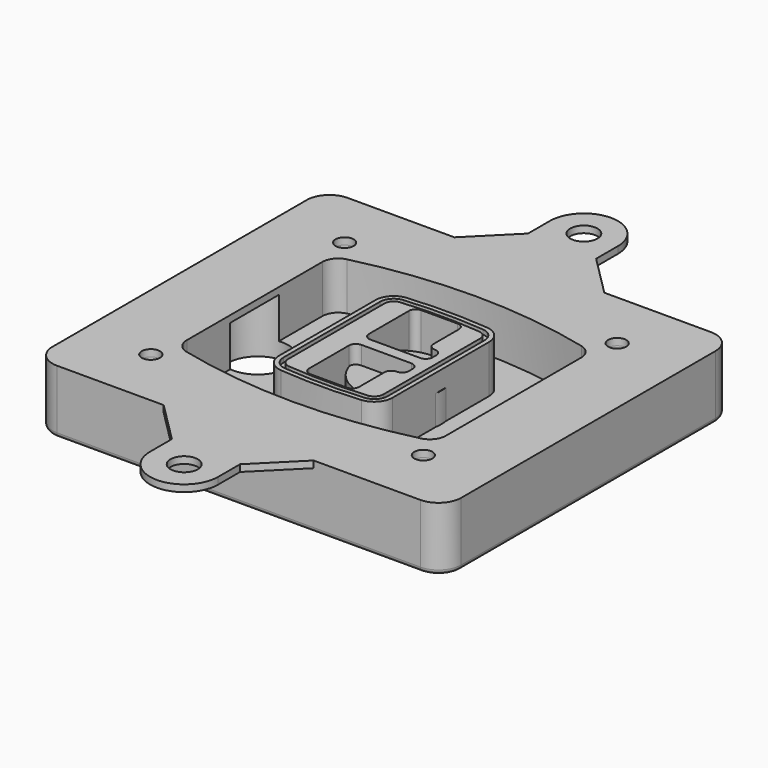
from build123d import *

# Parameters (mm, degrees)
F0_R      = 4
F1_DEPTH  = 25
F2_DEPTH  = 3
F3_DEPTH  = 18
F5_DEPTH  = 21
F6_DEPTH  = 2
F8_DEPTH  = 20
F9_DEPTH  = 16
F10_DEPTH = 25
F7_R      = 6
F7_R_2    = 4
F11_DEPTH = 6
F13_DEPTH = 9
F15_R     = 2
F16_R     = 4
F16_R_2   = 6
F17_DEPTH = 3


# Not quite as in the source:
# - a feature of the source that left no trace in its solid (it failed there, or was rolled back) is left out
# - a feature names something its author has since deleted; it is built from what else it names


with BuildPart() as f1:
    # F0 (on Top) → F1 (new body)
    with BuildSketch(Plane.XY):
        with BuildLine():
            ThreePointArc((-90, -70), (-87.0710678119, -77.0710678119), (-80, -80))
            Line((-80, -80), (80, -80))
            ThreePointArc((80, -80), (87.0710678119, -77.0710678119), (90, -70))
            Line((90, -70), (90, 70))
            ThreePointArc((90, 70), (87.0710678119, 77.0710678119), (80, 80))
            Line((80, 80), (-80, 80))
            ThreePointArc((-80, 80), (-87.0710678119, 77.0710678119), (-90, 70))
            Line((-90, 70), (-90, -70))
        make_face()
        with Locations((-60, -53.3333333333)):
            Circle(F0_R, mode=Mode.SUBTRACT)
        with Locations((60, -53.3333333333)):
            Circle(F0_R, mode=Mode.SUBTRACT)
        with Locations((-60, 53.3333333333)):
            Circle(F0_R, mode=Mode.SUBTRACT)
        with BuildLine():
            ThreePointArc((-64, 37.2990447398), (-61.0143011354, 45.9411029726), (-53.3306899286, 50.8970778549))
            ThreePointArc((-53.3306899286, 50.8970778549), (0, 57.3333333333), (53.3306899286, 50.8970778549))
            ThreePointArc((53.3306899286, 50.8970778549), (61.0143011354, 45.9411029726), (64, 37.2990447398))
            Line((64, 37.2990447398), (64, -37.2990447398))
            ThreePointArc((64, -37.2990447398), (61.0143011354, -45.9411029726), (53.3306899286, -50.8970778549))
            ThreePointArc((53.3306899286, -50.8970778549), (0, -57.3333333333), (-53.3306899286, -50.8970778549))
            ThreePointArc((-53.3306899286, -50.8970778549), (-61.0143011354, -45.9411029726), (-64, -37.2990447398))
            Line((-64, -37.2990447398), (-64, 37.2990447398))
        make_face(mode=Mode.SUBTRACT)
        with Locations((60, 53.3333333333)):
            Circle(F0_R, mode=Mode.SUBTRACT)
        with BuildLine():
            ThreePointArc((53.3306899286, 50.8970778549), (0, 57.3333333333), (-53.3306899286, 50.8970778549))
            ThreePointArc((-53.3306899286, 50.8970778549), (-61.0143011354, 45.9411029726), (-64, 37.2990447398))
            Line((-64, 37.2990447398), (-64, -37.2990447398))
            ThreePointArc((-64, -37.2990447398), (-61.0143011354, -45.9411029726), (-53.3306899286, -50.8970778549))
            ThreePointArc((-53.3306899286, -50.8970778549), (0, -57.3333333333), (53.3306899286, -50.8970778549))
            ThreePointArc((53.3306899286, -50.8970778549), (61.0143011354, -45.9411029726), (64, -37.2990447398))
            Line((64, -37.2990447398), (64, 37.2990447398))
            ThreePointArc((64, 37.2990447398), (61.0143011354, 45.9411029726), (53.3306899286, 50.8970778549))
        make_face()
        with BuildLine():
            Line((-60, -37.2990447398), (-60, 37.2990447398))
            ThreePointArc((-60, 37.2990447398), (-57.8673579538, 43.4719434775), (-52.3790642347, 47.0119255363))
            ThreePointArc((-52.3790642347, 47.0119255363), (0, 53.3333333333), (52.3790642347, 47.0119255363))
            ThreePointArc((52.3790642347, 47.0119255363), (57.8673579538, 43.4719434775), (60, 37.2990447398))
            Line((60, 37.2990447398), (60, -37.2990447398))
            ThreePointArc((60, -37.2990447398), (57.8673579538, -43.4719434775), (52.3790642347, -47.0119255363))
            ThreePointArc((52.3790642347, -47.0119255363), (0, -53.3333333333), (-52.3790642347, -47.0119255363))
            ThreePointArc((-52.3790642347, -47.0119255363), (-57.8673579538, -43.4719434775), (-60, -37.2990447398))
        make_face(mode=Mode.SUBTRACT)
        with BuildLine():
            ThreePointArc((-52.3790642347, 47.0119255363), (-57.8673579538, 43.4719434775), (-60, 37.2990447398))
            Line((-60, 37.2990447398), (-60, -37.2990447398))
            ThreePointArc((-60, -37.2990447398), (-57.8673579538, -43.4719434775), (-52.3790642347, -47.0119255363))
            ThreePointArc((-52.3790642347, -47.0119255363), (0, -53.3333333333), (52.3790642347, -47.0119255363))
            ThreePointArc((52.3790642347, -47.0119255363), (57.8673579538, -43.4719434775), (60, -37.2990447398))
            Line((60, -37.2990447398), (60, 37.2990447398))
            ThreePointArc((60, 37.2990447398), (57.8673579538, 43.4719434775), (52.3790642347, 47.0119255363))
            ThreePointArc((52.3790642347, 47.0119255363), (0, 53.3333333333), (-52.3790642347, 47.0119255363))
        make_face()
        with BuildLine():
            ThreePointArc((51.6653449643, 44.0980612973), (55.5071505677, 41.6200738562), (57, 37.2990447398))
            Line((57, 37.2990447398), (57, -37.2990447398))
            ThreePointArc((57, -37.2990447398), (55.5071505677, -41.6200738562), (51.6653449643, -44.0980612973))
            ThreePointArc((51.6653449643, -44.0980612973), (0, -50.3333333333), (-51.6653449643, -44.0980612973))
            ThreePointArc((-51.6653449643, -44.0980612973), (-55.5071505677, -41.6200738562), (-57, -37.2990447398))
            Line((-57, -37.2990447398), (-57, 37.2990447398))
            ThreePointArc((-57, 37.2990447398), (-55.5071505677, 41.6200738562), (-51.6653449643, 44.0980612973))
            ThreePointArc((-51.6653449643, 44.0980612973), (0, 50.3333333333), (51.6653449643, 44.0980612973))
        make_face(mode=Mode.SUBTRACT)
        with BuildLine():
            Line((57, -37.2990447398), (57, 37.2990447398))
            ThreePointArc((57, 37.2990447398), (55.5071505677, 41.6200738562), (51.6653449643, 44.0980612973))
            ThreePointArc((51.6653449643, 44.0980612973), (0, 50.3333333333), (-51.6653449643, 44.0980612973))
            ThreePointArc((-51.6653449643, 44.0980612973), (-55.5071505677, 41.6200738562), (-57, 37.2990447398))
            Line((-57, 37.2990447398), (-57, -37.2990447398))
            ThreePointArc((-57, -37.2990447398), (-55.5071505677, -41.6200738562), (-51.6653449643, -44.0980612973))
            ThreePointArc((-51.6653449643, -44.0980612973), (0, -50.3333333333), (51.6653449643, -44.0980612973))
            ThreePointArc((51.6653449643, -44.0980612973), (55.5071505677, -41.6200738562), (57, -37.2990447398))
        make_face()
    extrude(amount=-F1_DEPTH)

    # F0 (on Top) → F2 (join)
    with BuildSketch(Plane.XY):
        with BuildLine():
            ThreePointArc((-52.3790642347, 47.0119255363), (-57.8673579538, 43.4719434775), (-60, 37.2990447398))
            Line((-60, 37.2990447398), (-60, -37.2990447398))
            ThreePointArc((-60, -37.2990447398), (-57.8673579538, -43.4719434775), (-52.3790642347, -47.0119255363))
            ThreePointArc((-52.3790642347, -47.0119255363), (0, -53.3333333333), (52.3790642347, -47.0119255363))
            ThreePointArc((52.3790642347, -47.0119255363), (57.8673579538, -43.4719434775), (60, -37.2990447398))
            Line((60, -37.2990447398), (60, 37.2990447398))
            ThreePointArc((60, 37.2990447398), (57.8673579538, 43.4719434775), (52.3790642347, 47.0119255363))
            ThreePointArc((52.3790642347, 47.0119255363), (0, 53.3333333333), (-52.3790642347, 47.0119255363))
        make_face()
        with BuildLine():
            ThreePointArc((51.6653449643, 44.0980612973), (55.5071505677, 41.6200738562), (57, 37.2990447398))
            Line((57, 37.2990447398), (57, -37.2990447398))
            ThreePointArc((57, -37.2990447398), (55.5071505677, -41.6200738562), (51.6653449643, -44.0980612973))
            ThreePointArc((51.6653449643, -44.0980612973), (0, -50.3333333333), (-51.6653449643, -44.0980612973))
            ThreePointArc((-51.6653449643, -44.0980612973), (-55.5071505677, -41.6200738562), (-57, -37.2990447398))
            Line((-57, -37.2990447398), (-57, 37.2990447398))
            ThreePointArc((-57, 37.2990447398), (-55.5071505677, 41.6200738562), (-51.6653449643, 44.0980612973))
            ThreePointArc((-51.6653449643, 44.0980612973), (0, 50.3333333333), (51.6653449643, 44.0980612973))
        make_face(mode=Mode.SUBTRACT)
    extrude(amount=F2_DEPTH)

    # F0 (on Top) → F3 (cut)
    with BuildSketch(Plane.XY):
        with BuildLine():
            Line((57, -37.2990447398), (57, 37.2990447398))
            ThreePointArc((57, 37.2990447398), (55.5071505677, 41.6200738562), (51.6653449643, 44.0980612973))
            ThreePointArc((51.6653449643, 44.0980612973), (0, 50.3333333333), (-51.6653449643, 44.0980612973))
            ThreePointArc((-51.6653449643, 44.0980612973), (-55.5071505677, 41.6200738562), (-57, 37.2990447398))
            Line((-57, 37.2990447398), (-57, -37.2990447398))
            ThreePointArc((-57, -37.2990447398), (-55.5071505677, -41.6200738562), (-51.6653449643, -44.0980612973))
            ThreePointArc((-51.6653449643, -44.0980612973), (0, -50.3333333333), (51.6653449643, -44.0980612973))
            ThreePointArc((51.6653449643, -44.0980612973), (55.5071505677, -41.6200738562), (57, -37.2990447398))
        make_face()
    extrude(amount=-F3_DEPTH, mode=Mode.SUBTRACT)

    # F4 (on face) → F5 (join, through all)
    with BuildSketch(Plane.XY.offset(3)):
        with BuildLine():
            ThreePointArc((-25, -26.587695628), (-22.8992979869, -31.9912392117), (-17.7004291845, -34.5569740744))
            ThreePointArc((-17.7004291845, -34.5569740744), (0, -35.3333333333), (17.7004291845, -34.5569740744))
            ThreePointArc((17.7004291845, -34.5569740744), (22.8992979869, -31.9912392117), (25, -26.587695628))
            Line((25, -26.587695628), (25, 26.587695628))
            ThreePointArc((25, 26.587695628), (22.8992979869, 31.9912392117), (17.7004291845, 34.5569740744))
            ThreePointArc((17.7004291845, 34.5569740744), (0, 35.3333333333), (-17.7004291845, 34.5569740744))
            ThreePointArc((-17.7004291845, 34.5569740744), (-22.8992979869, 31.9912392117), (-25, 26.587695628))
            Line((-25, 26.587695628), (-25, -26.587695628))
        make_face()
        with BuildLine():
            ThreePointArc((17.5253218884, 32.5646544628), (21.4244734902, 30.6403533158), (23, 26.587695628))
            Line((23, 26.587695628), (23, -26.587695628))
            ThreePointArc((23, -26.587695628), (21.4244734902, -30.6403533158), (17.5253218884, -32.5646544628))
            ThreePointArc((17.5253218884, -32.5646544628), (0, -33.3333333333), (-17.5253218884, -32.5646544628))
            ThreePointArc((-17.5253218884, -32.5646544628), (-21.4244734902, -30.6403533158), (-23, -26.587695628))
            Line((-23, -26.587695628), (-23, 26.587695628))
            ThreePointArc((-23, 26.587695628), (-21.4244734902, 30.6403533158), (-17.5253218884, 32.5646544628))
            ThreePointArc((-17.5253218884, 32.5646544628), (0, 33.3333333333), (17.5253218884, 32.5646544628))
        make_face(mode=Mode.SUBTRACT)
        with BuildLine():
            Line((23, -26.587695628), (23, 26.587695628))
            ThreePointArc((23, 26.587695628), (21.4244734902, 30.6403533158), (17.5253218884, 32.5646544628))
            ThreePointArc((17.5253218884, 32.5646544628), (0, 33.3333333333), (-17.5253218884, 32.5646544628))
            ThreePointArc((-17.5253218884, 32.5646544628), (-21.4244734902, 30.6403533158), (-23, 26.587695628))
            Line((-23, 26.587695628), (-23, -26.587695628))
            ThreePointArc((-23, -26.587695628), (-21.4244734902, -30.6403533158), (-17.5253218884, -32.5646544628))
            ThreePointArc((-17.5253218884, -32.5646544628), (0, -33.3333333333), (17.5253218884, -32.5646544628))
            ThreePointArc((17.5253218884, -32.5646544628), (21.4244734902, -30.6403533158), (23, -26.587695628))
        make_face()
        with BuildLine():
            ThreePointArc((17.3502145923, 30.5723348512), (19.9496489934, 29.2894674198), (21, 26.587695628))
            Line((21, 26.587695628), (21, -26.587695628))
            ThreePointArc((21, -26.587695628), (19.9496489934, -29.2894674198), (17.3502145923, -30.5723348512))
            ThreePointArc((17.3502145923, -30.5723348512), (0, -31.3333333333), (-17.3502145923, -30.5723348512))
            ThreePointArc((-17.3502145923, -30.5723348512), (-19.9496489934, -29.2894674198), (-21, -26.587695628))
            Line((-21, -26.587695628), (-21, 26.587695628))
            ThreePointArc((-21, 26.587695628), (-19.9496489934, 29.2894674198), (-17.3502145923, 30.5723348512))
            ThreePointArc((-17.3502145923, 30.5723348512), (0, 31.3333333333), (17.3502145923, 30.5723348512))
        make_face(mode=Mode.SUBTRACT)
        with BuildLine():
            Line((21, -26.587695628), (21, 26.587695628))
            ThreePointArc((21, 26.587695628), (19.9496489934, 29.2894674198), (17.3502145923, 30.5723348512))
            ThreePointArc((17.3502145923, 30.5723348512), (0, 31.3333333333), (-17.3502145923, 30.5723348512))
            ThreePointArc((-17.3502145923, 30.5723348512), (-19.9496489934, 29.2894674198), (-21, 26.587695628))
            Line((-21, 26.587695628), (-21, -26.587695628))
            ThreePointArc((-21, -26.587695628), (-19.9496489934, -29.2894674198), (-17.3502145923, -30.5723348512))
            ThreePointArc((-17.3502145923, -30.5723348512), (0, -31.3333333333), (17.3502145923, -30.5723348512))
            ThreePointArc((17.3502145923, -30.5723348512), (19.9496489934, -29.2894674198), (21, -26.587695628))
        make_face()
        with BuildLine():
            Line((-8, -2.5), (14, -2.5))
            ThreePointArc((14, -2.5), (16.1213203436, -3.3786796564), (17, -5.5))
            Line((17, -5.5), (17, -7.5))
            ThreePointArc((17, -7.5), (16.1213203436, -9.6213203436), (14, -10.5))
            ThreePointArc((14, -10.5), (11.8786796564, -11.3786796564), (11, -13.5))
            Line((11, -13.5), (11, -27.5))
            ThreePointArc((11, -27.5), (10.1213203436, -29.6213203436), (8, -30.5))
            Line((8, -30.5), (-8, -30.5))
            ThreePointArc((-8, -30.5), (-10.1213203436, -29.6213203436), (-11, -27.5))
            Line((-11, -27.5), (-11, -5.5))
            ThreePointArc((-11, -5.5), (-10.1213203436, -3.3786796564), (-8, -2.5))
        make_face(mode=Mode.SUBTRACT)
        with BuildLine():
            ThreePointArc((-8, 2.5), (-10.1213203436, 3.3786796564), (-11, 5.5))
            Line((-11, 5.5), (-11, 27.5))
            ThreePointArc((-11, 27.5), (-10.1213203436, 29.6213203436), (-8, 30.5))
            Line((-8, 30.5), (8, 30.5))
            ThreePointArc((8, 30.5), (10.1213203436, 29.6213203436), (11, 27.5))
            Line((11, 27.5), (11, 13.5))
            ThreePointArc((11, 13.5), (11.8786796564, 11.3786796564), (14, 10.5))
            ThreePointArc((14, 10.5), (16.1213203436, 9.6213203436), (17, 7.5))
            Line((17, 7.5), (17, 5.5))
            ThreePointArc((17, 5.5), (16.1213203436, 3.3786796564), (14, 2.5))
            Line((14, 2.5), (-8, 2.5))
        make_face(mode=Mode.SUBTRACT)
    extrude(amount=-F5_DEPTH)

    # F4 (on face) → F6 (cut)
    with BuildSketch(Plane.XY.offset(3)):
        with BuildLine():
            Line((23, -26.587695628), (23, 26.587695628))
            ThreePointArc((23, 26.587695628), (21.4244734902, 30.6403533158), (17.5253218884, 32.5646544628))
            ThreePointArc((17.5253218884, 32.5646544628), (0, 33.3333333333), (-17.5253218884, 32.5646544628))
            ThreePointArc((-17.5253218884, 32.5646544628), (-21.4244734902, 30.6403533158), (-23, 26.587695628))
            Line((-23, 26.587695628), (-23, -26.587695628))
            ThreePointArc((-23, -26.587695628), (-21.4244734902, -30.6403533158), (-17.5253218884, -32.5646544628))
            ThreePointArc((-17.5253218884, -32.5646544628), (0, -33.3333333333), (17.5253218884, -32.5646544628))
            ThreePointArc((17.5253218884, -32.5646544628), (21.4244734902, -30.6403533158), (23, -26.587695628))
        make_face()
        with BuildLine():
            ThreePointArc((17.3502145923, 30.5723348512), (19.9496489934, 29.2894674198), (21, 26.587695628))
            Line((21, 26.587695628), (21, -26.587695628))
            ThreePointArc((21, -26.587695628), (19.9496489934, -29.2894674198), (17.3502145923, -30.5723348512))
            ThreePointArc((17.3502145923, -30.5723348512), (0, -31.3333333333), (-17.3502145923, -30.5723348512))
            ThreePointArc((-17.3502145923, -30.5723348512), (-19.9496489934, -29.2894674198), (-21, -26.587695628))
            Line((-21, -26.587695628), (-21, 26.587695628))
            ThreePointArc((-21, 26.587695628), (-19.9496489934, 29.2894674198), (-17.3502145923, 30.5723348512))
            ThreePointArc((-17.3502145923, 30.5723348512), (0, 31.3333333333), (17.3502145923, 30.5723348512))
        make_face(mode=Mode.SUBTRACT)
    extrude(amount=-F6_DEPTH, mode=Mode.SUBTRACT)

    # F7 (on face) → F8 (join)
    with BuildSketch(Plane(origin=(0, 0, -25), x_dir=(1, 0, 0), z_dir=(0, 0, -1))):
        with BuildLine():
            ThreePointArc((-6.71157564, 0), (6.7567035675, 13.4682792075), (20.224982775, 0))
            Line((20.224982775, 0), (25.224982775, 0))
            ThreePointArc((25.224982775, 0), (6.7567035675, 18.4682792075), (-11.71157564, 0))
            Line((-11.71157564, 0), (-6.71157564, 0))
        make_face()
        with BuildLine():
            Line((-6.71157564, 0), (20.224982775, 0))
            ThreePointArc((20.224982775, 0), (6.7567035675, 13.4682792075), (-6.71157564, 0))
        make_face()
        with BuildLine():
            ThreePointArc((-6.71157564, 0), (6.7567035675, -13.4682792075), (20.224982775, 0))
            Line((20.224982775, 0), (-6.71157564, 0))
        make_face()
        with BuildLine():
            Line((25.224982775, 0), (20.224982775, 0))
            ThreePointArc((20.224982775, 0), (6.7567035675, -13.4682792075), (-6.71157564, 0))
            Line((-6.71157564, 0), (-11.71157564, 0))
            ThreePointArc((-11.71157564, 0), (6.7567035675, -18.4682792075), (25.224982775, 0))
        make_face()
    extrude(amount=-F8_DEPTH)

    # F7 (on face) → F9 (cut)
    with BuildSketch(Plane(origin=(0, 0, -25), x_dir=(1, 0, 0), z_dir=(0, 0, -1))):
        with BuildLine():
            Line((-6.71157564, 0), (20.224982775, 0))
            ThreePointArc((20.224982775, 0), (6.7567035675, 13.4682792075), (-6.71157564, 0))
        make_face()
        with BuildLine():
            ThreePointArc((-6.71157564, 0), (6.7567035675, -13.4682792075), (20.224982775, 0))
            Line((20.224982775, 0), (-6.71157564, 0))
        make_face()
    extrude(amount=-F9_DEPTH, mode=Mode.SUBTRACT)

    # F7 (on face) → F10 (cut)
    with BuildSketch(Plane(origin=(0, 0, -25), x_dir=(1, 0, 0), z_dir=(0, 0, -1))):
        with BuildLine():
            Line((-69.0318229325, 0), (-42.0952645175, 0))
            ThreePointArc((-42.0952645175, 0), (-55.563543725, 13.4682792075), (-69.0318229325, 0))
        make_face()
        with BuildLine():
            ThreePointArc((-69.0318229325, 0), (-55.563543725, -13.4682792075), (-42.0952645175, 0))
            Line((-42.0952645175, 0), (-69.0318229325, 0))
        make_face()
    extrude(amount=-F10_DEPTH, mode=Mode.SUBTRACT)

    # F7 (on face) → F11 (cut)
    with BuildSketch(Plane(origin=(0, 0, -25), x_dir=(1, 0, 0), z_dir=(0, 0, -1))):
        with Locations((60, -53.3333333333)):
            Circle(F7_R)
        with Locations((60, -53.3333333333)):
            Circle(F7_R_2, mode=Mode.SUBTRACT)
        with Locations((-60, -53.3333333333)):
            Circle(F7_R)
        with Locations((-60, -53.3333333333)):
            Circle(F7_R_2, mode=Mode.SUBTRACT)
        with Locations((-60, 53.3333333333)):
            Circle(F7_R)
        with Locations((-60, 53.3333333333)):
            Circle(F7_R_2, mode=Mode.SUBTRACT)
        with Locations((60, 53.3333333333)):
            Circle(F7_R)
        with Locations((60, 53.3333333333)):
            Circle(F7_R_2, mode=Mode.SUBTRACT)
    extrude(amount=-F11_DEPTH, mode=Mode.SUBTRACT)

    # F12 (on face) → F13 (cut, through all)
    with BuildSketch(Plane(origin=(0, 0, -9), x_dir=(1, 0, 0), z_dir=(0, 0, -1))):
        with BuildLine():
            ThreePointArc((20.224982775, 0), (20.1663399806, 1.2554664788), (19.9909222755, 2.5))
            Line((19.9909222755, 2.5), (14, 2.5))
            ThreePointArc((14, 2.5), (16.1213203436, 3.3786796564), (17, 5.5))
            Line((17, 5.5), (17, 7.5))
            ThreePointArc((17, 7.5), (16.1213203436, 9.6213203436), (14, 10.5))
            ThreePointArc((14, 10.5), (12.1627255951, 11.1284134507), (11.0951631559, 12.750384826))
            ThreePointArc((11.0951631559, 12.750384826), (11.0476113807, 12.7664660322), (11, 12.7823698976))
            Line((11, 12.7823698976), (11, -12.7823698976))
            ThreePointArc((11, -12.7823698976), (11.0476113807, -12.7664660322), (11.0951631559, -12.750384826))
            ThreePointArc((11.0951631559, -12.750384826), (12.1627255951, -11.1284134507), (14, -10.5))
            ThreePointArc((14, -10.5), (16.1213203436, -9.6213203436), (17, -7.5))
            Line((17, -7.5), (17, -5.5))
            ThreePointArc((17, -5.5), (16.1213203436, -3.3786796564), (14, -2.5))
            Line((14, -2.5), (19.9909222755, -2.5))
            ThreePointArc((19.9909222755, -2.5), (20.1663399806, -1.2554664788), (20.224982775, 0))
        make_face()
    extrude(amount=F13_DEPTH, mode=Mode.SUBTRACT)

    # F15
    f15_edges = [f1.edges().sort_by_distance(p)[0] for p in [
        (0, -80, -25),
        (-87.071068, -77.071068, -25),
        (-90, 0, -25),
        (-87.071068, 77.071068, -25),
        (87.071068, -77.071068, -25),
        (0, 80, -25),
        (90, 0, -25),
        (87.071068, 77.071068, -25),
    ]]
    fillet(f15_edges, radius=F15_R)

    # F16 (on face) → F17 (join, through all)
    with BuildSketch(Plane.XY):
        with BuildLine():
            Line((-90, 70), (-90, -70))
            ThreePointArc((-90, -70), (-87.0710678119, -77.0710678119), (-80, -80))
            Line((-80, -80), (-33, -80))
            Line((-33, -80), (33, -80))
            Line((33, -80), (80, -80))
            ThreePointArc((80, -80), (87.0710678119, -77.0710678119), (90, -70))
            Line((90, -70), (90, 70))
            ThreePointArc((90, 70), (87.0710678119, 77.0710678119), (80, 80))
            Line((80, 80), (33, 80))
            Line((33, 80), (-33, 80))
            Line((-33, 80), (-80, 80))
            ThreePointArc((-80, 80), (-87.0710678119, 77.0710678119), (-90, 70))
        make_face()
        with Locations((-60, -53.3333333333)):
            Circle(F16_R, mode=Mode.SUBTRACT)
        with Locations((60, -53.3333333333)):
            Circle(F16_R, mode=Mode.SUBTRACT)
        with Locations((-60, 53.3333333333)):
            Circle(F16_R, mode=Mode.SUBTRACT)
        with BuildLine():
            Line((-60, -37.2990447398), (-60, 37.2990447398))
            ThreePointArc((-60, 37.2990447398), (-57.8673579538, 43.4719434775), (-52.3790642347, 47.0119255363))
            ThreePointArc((-52.3790642347, 47.0119255363), (0, 53.3333333333), (52.3790642347, 47.0119255363))
            ThreePointArc((52.3790642347, 47.0119255363), (57.8673579538, 43.4719434775), (60, 37.2990447398))
            Line((60, 37.2990447398), (60, -37.2990447398))
            ThreePointArc((60, -37.2990447398), (57.8673579538, -43.4719434775), (52.3790642347, -47.0119255363))
            ThreePointArc((52.3790642347, -47.0119255363), (0, -53.3333333333), (-52.3790642347, -47.0119255363))
            ThreePointArc((-52.3790642347, -47.0119255363), (-57.8673579538, -43.4719434775), (-60, -37.2990447398))
        make_face(mode=Mode.SUBTRACT)
        with Locations((60, 53.3333333333)):
            Circle(F16_R, mode=Mode.SUBTRACT)
        with BuildLine():
            Line((33, -80), (-33, -80))
            Line((-33, -80), (-15, -98))
            Line((-15, -98), (-15, -110))
            ThreePointArc((-15, -110), (0, -125), (15, -110))
            Line((15, -110), (15, -98))
            Line((15, -98), (33, -80))
        make_face()
        with Locations((0, -110)):
            Circle(F16_R_2, mode=Mode.SUBTRACT)
        with BuildLine():
            Line((-15, 98), (-33, 80))
            Line((-33, 80), (33, 80))
            Line((33, 80), (15, 98))
            Line((15, 98), (15, 110))
            ThreePointArc((15, 110), (0, 125), (-15, 110))
            Line((-15, 110), (-15, 98))
        make_face()
        with Locations((0, 110)):
            Circle(F16_R_2, mode=Mode.SUBTRACT)
    extrude(amount=F17_DEPTH)


solid = f1.part
